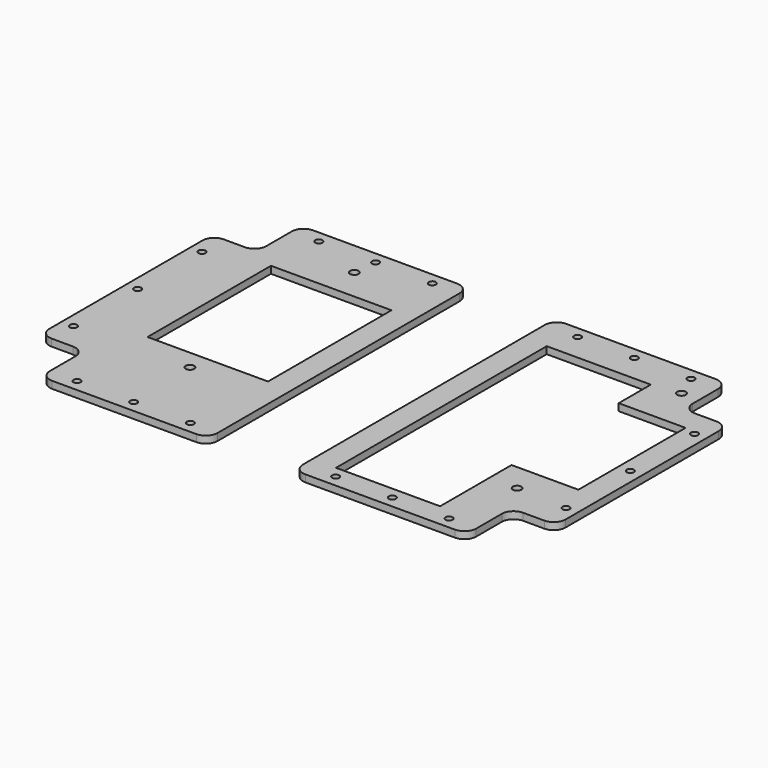
from build123d import *

# Parameters (mm, degrees)
F0_W      = 90
F0_H      = 138
F0_R      = 1.5
F1_DEPTH  = 3
F0_W_2    = 92.3638074994
F2_W      = 19
F2_H      = 23.5
F3_DEPTH  = 25
F4_W      = 19
F4_H      = 23.5
F5_DEPTH  = 25
F6_R      = 5
F6_2_R    = 5
F7_R      = 1.8
F8_DEPTH  = 25
F9_W      = 28.3
F9_H      = 56.7
F10_DEPTH = 25
F11_W     = 51
F11_H     = 65.3
F12_DEPTH = 25


# Not quite as in the source:
# - a feature names something its author has since deleted; it is built from what else it names


with BuildPart() as f1:
    # F0 (on Top) → F1 (new body)
    with BuildSketch(Plane.XY):
        with Locations((-9.5, 0)):
            Rectangle(F0_W, F0_H)
        with Locations((-24, -64)):
            Circle(F0_R, mode=Mode.SUBTRACT)
        with Locations((0, -64)):
            Circle(F0_R, mode=Mode.SUBTRACT)
        with Locations((24, -64)):
            Circle(F0_R, mode=Mode.SUBTRACT)
        with Locations((-49.5, -34)):
            Circle(F0_R, mode=Mode.SUBTRACT)
        with Locations((-49.5, 0)):
            Circle(F0_R, mode=Mode.SUBTRACT)
        with Locations((-49.5, 34)):
            Circle(F0_R, mode=Mode.SUBTRACT)
        with Locations((-24, 64)):
            Circle(F0_R, mode=Mode.SUBTRACT)
        with Locations((0, 64)):
            Circle(F0_R, mode=Mode.SUBTRACT)
        with Locations((24, 64)):
            Circle(F0_R, mode=Mode.SUBTRACT)
    extrude(amount=F1_DEPTH)

    # F2 (on face) → F3 (cut)
    with BuildSketch(Plane.XY.offset(3)):
        with Locations((-45, 57.25)):
            Rectangle(F2_W, F2_H)
        with Locations((-45, -57.25)):
            Rectangle(F2_W, F2_H)
    extrude(amount=-F3_DEPTH, mode=Mode.SUBTRACT)

    # F6
    f6_edges = [f1.edges().sort_by_distance(p)[0] for p in [
        (-54.5, 45.5, 1.5),
        (-54.5, -45.5, 1.5),
        (-35.5, -45.5, 1.5),
        (-35.5, -69, 1.5),
        (35.5, -69, 1.5),
        (35.5, 69, 1.5),
        (-35.5, 69, 1.5),
        (-35.5, 45.5, 1.5),
    ]]
    fillet(f6_edges, radius=F6_R)


with BuildPart() as f1b:
    # F0 (on Top) → F1, piece 2 (new body)
    with BuildSketch(Plane.XY):
        with Locations((117.8180962503, 0)):
            Rectangle(F0_W_2, F0_H)
        with Locations((85.5, -64)):
            Circle(F0_R, mode=Mode.SUBTRACT)
        with Locations((109.5, -64)):
            Circle(F0_R, mode=Mode.SUBTRACT)
        with Locations((133.5, -64)):
            Circle(F0_R, mode=Mode.SUBTRACT)
        with Locations((159, -34)):
            Circle(F0_R, mode=Mode.SUBTRACT)
        with Locations((159, 0)):
            Circle(F0_R, mode=Mode.SUBTRACT)
        with Locations((159, 34)):
            Circle(F0_R, mode=Mode.SUBTRACT)
        with Locations((85.5, 64)):
            Circle(F0_R, mode=Mode.SUBTRACT)
        with Locations((109.5, 64)):
            Circle(F0_R, mode=Mode.SUBTRACT)
        with Locations((133.5, 64)):
            Circle(F0_R, mode=Mode.SUBTRACT)
    extrude(amount=F1_DEPTH)

    # F4 (on face) → F5 (cut)
    with BuildSketch(Plane.XY.offset(3)):
        with Locations((154.5, 57.25)):
            Rectangle(F4_W, F4_H)
        with Locations((154.5, -57.25)):
            Rectangle(F4_W, F4_H)
    extrude(amount=-F5_DEPTH, mode=Mode.SUBTRACT)

    # F6#2
    f6_2_edges = [f1b.edges().sort_by_distance(p)[0] for p in [
        (71.636193, 69, 1.5),
        (145, 69, 1.5),
        (145, 45.5, 1.5),
        (164, 45.5, 1.5),
        (164, -45.5, 1.5),
        (145, -45.5, 1.5),
        (145, -69, 1.5),
        (71.636193, -69, 1.5),
    ]]
    fillet(f6_2_edges, radius=F6_2_R)


with BuildPart() as f8_tool:
    # F7 (on face) → F8 (new body)
    with BuildSketch(Plane.XY.offset(3)):
        with Locations((-1, 54)):
            Circle(F7_R)
        with Locations((-1, -33)):
            Circle(F7_R)
        with Locations((137.5, -33)):
            Circle(F7_R)
        with Locations((137.5, 54)):
            Circle(F7_R)
    extrude(amount=-F8_DEPTH)


with BuildPart() as f1_1:
    add(f1.part)

    # F8: cut by f8_tool
    add(f8_tool.part, mode=Mode.SUBTRACT)

    # F11 (on face) → F12 (cut)
    with BuildSketch(Plane.XY.offset(3)):
        with Locations((0, 7.85)):
            Rectangle(F11_W, F11_H)
    extrude(amount=-F12_DEPTH, mode=Mode.SUBTRACT)


with BuildPart() as f1b_1:
    add(f1b.part)

    # F8: cut by f8_tool
    add(f8_tool.part, mode=Mode.SUBTRACT)

    # F9 (on face) → F10 (cut)
    with BuildSketch(Plane.XY.offset(3)):
        Polygon((125.7, 52.5), (81.6361925006, 52.5), (81.6361925006, -59), (125.7, -59), (125.7, -21.2), (125.7, 35.5), align=None)
        with Locations((139.85, 7.15)):
            Rectangle(F9_W, F9_H)
    extrude(amount=-F10_DEPTH, mode=Mode.SUBTRACT)


solid = Compound([f1_1.part, f1b_1.part])
